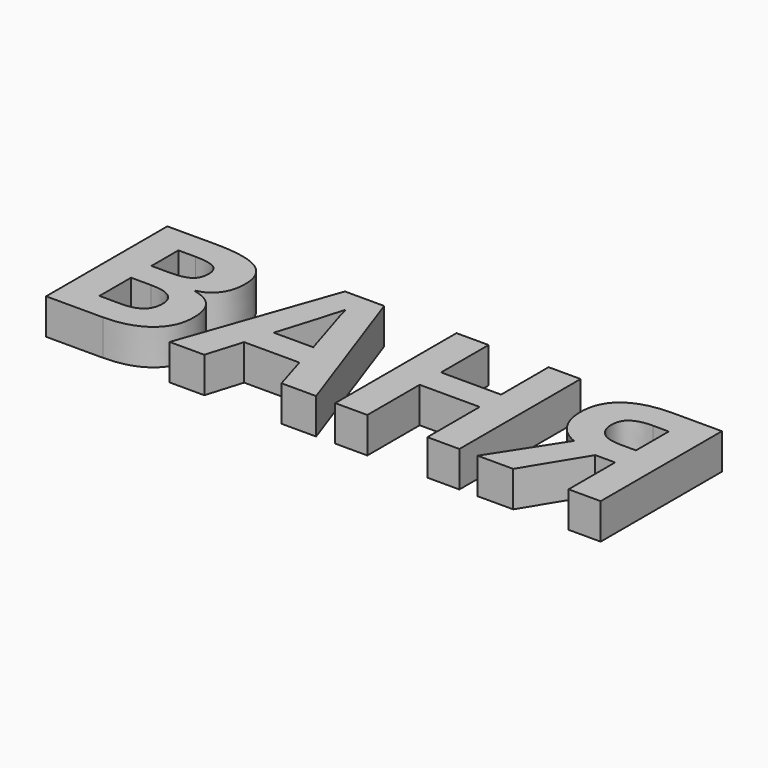
from build123d import *

# Parameters (mm, degrees)
F0_TEXT_SIZE = 41.6666666667
F1_DEPTH     = 7


# Not quite as in the source:
# - Text() gives the source's letters only with a copy of the font that has no kerning and outlines rounded to 1/6400 em; it was checked with that copy


with BuildPart() as f1:
    # F0 (on Top) → F1 (new body)
    with BuildSketch(Plane.XY):
        with Locations((-33.2492585692, -15.1780416865)):
            Text('ВАНЯ', F0_TEXT_SIZE, font='Open Sans', font_style=FontStyle.BOLD, text_align=(TextAlign.LEFT, TextAlign.BOTTOM))
    extrude(amount=F1_DEPTH)


solid = f1.part
